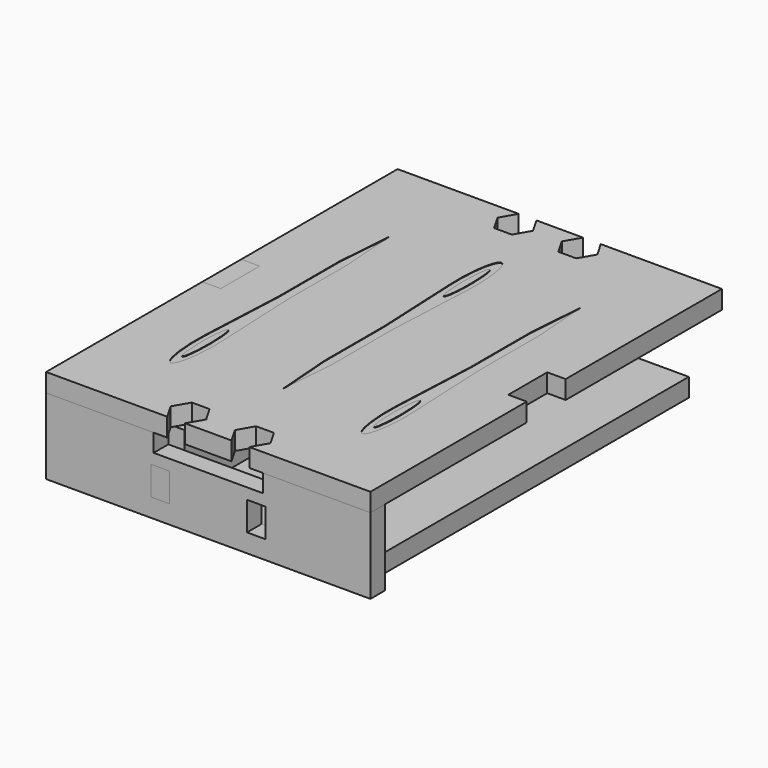
from build123d import *

# Parameters (mm, degrees)
F1_W      = 50
F1_H      = 70
F1_W_2    = 3.2
F1_H_2    = 23.3333333333
F2_DEPTH  = 3.2
F4_DEPTH  = 3.2
F6_DEPTH  = 3.2
F8_DEPTH  = 3.2
F10_DEPTH = 3.2
F11_W     = 18.7
F11_H     = 3.2
F12_DEPTH = 3.2
F14_DEPTH = 0.1
F16_DEPTH = 3.2


# Not quite as in the source:
# - a feature names something its author has since deleted; it is built from what else it names


with BuildPart() as f2:
    # F1 (on Top) → F2 (new body)
    with BuildSketch(Plane.XY):
        Rectangle(F1_W, F1_H)
        with Locations((-8.3333333333, 0)):
            Rectangle(F1_W_2, F1_H_2, mode=Mode.SUBTRACT)
        with Locations((8.3333333333, 0)):
            Rectangle(F1_W_2, F1_H_2, mode=Mode.SUBTRACT)
    extrude(amount=F2_DEPTH)


with BuildPart() as f4:
    # F3 (on face) → F4 (new body)
    with BuildSketch(Plane(origin=(-25, 0, 0), x_dir=(0, -1, 0), z_dir=(-1, 0, 0))):
        Polygon((-35, 13.2), (-35, 0), (35, 0), (35, 13.2), (14.2401693586, 13.2), (8.4666666667, 3.2), (-8.4666666667, 3.2), (-14.2401693586, 13.2), align=None)
    extrude(amount=F4_DEPTH)


with BuildPart() as f6:
    # F5 (on face) → F6 (new body)
    with BuildSketch(Plane(origin=(-6.7333333333, 0, 0), x_dir=(0, -1, 0), z_dir=(-1, 0, 0))):
        Polygon((38.2, 3.2), (38.2, 8.2), (35, 8.2), (35, 13.2), (14.2401693586, 13.2), (8.4666666667, 3.2), (11.6666666667, 3.2), (35, 3.2), align=None)
        Polygon((-8.4666666667, 3.2), (-14.2401693586, 13.2), (-35, 13.2), (-35, 8.2), (-38.2, 8.2), (-38.2, 3.2), (-35, 3.2), (-11.6666666667, 3.2), align=None)
        Polygon((11.6666666667, 0), (11.6666666667, 3.2), (8.4666666667, 3.2), (-8.4666666667, 3.2), (-11.6666666667, 3.2), (-11.6666666667, 0), align=None)
    extrude(amount=F6_DEPTH)


with BuildPart() as f8:
    # F7 (on face) → F8 (new body)
    with BuildSketch(Plane.XZ.offset(35)):
        Polygon((25, 3.2), (25, 0), (28.2, 0), (28.2, 13.2), (25, 13.2), align=None)
        Polygon((-25, 3.2), (-25, 0), (25, 0), (25, 3.2), (9.9333333333, 3.2), (6.7333333333, 3.2), (-6.7333333333, 3.2), (-9.9333333333, 3.2), align=None)
        Polygon((-28.2, 13.2), (-28.2, 0), (-25, 0), (-25, 3.2), (-9.9333333333, 3.2), (-9.9333333333, 8.2), (-6.7333333333, 8.2), (-6.7333333333, 3.2), (6.7333333333, 3.2), (6.7333333333, 8.2), (9.9333333333, 8.2), (9.9333333333, 3.2), (25, 3.2), (25, 13.2), (9.5, 13.2), (9.5, 10.1), (-9.5, 10.1), (-9.5, 13.2), align=None)
    extrude(amount=F8_DEPTH)


with BuildPart() as f10:
    # F9 (on face) → F10 (new body)
    with BuildSketch(Plane(origin=(-28.2, 0, 0), x_dir=(0, -1, 0), z_dir=(-1, 0, 0))):
        Polygon((-14.2401693586, 13.2), (-8.4666666667, 3.2), (8.4666666667, 3.2), (14.2401693586, 13.2), (4.2333333333, 13.2), (4.2333333333, 16.4), (-4.2333333333, 16.4), (-4.2333333333, 13.2), align=None)
    extrude(amount=-F10_DEPTH)


with BuildPart() as f12:
    # F11 (on face) → F12 (new body)
    with BuildSketch(Plane.XY.offset(13.2)):
        Polygon((-28.2, 38.2), (-28.2, 4.2333333333), (-25, 4.2333333333), (-25, -4.2333333333), (-28.2, -4.2333333333), (-28.2, -35), (-9.5, -35), (-9.5, -38.2), (-7.1332359102, -38.2), (-8.6776478803, -35.525), (-7.1332359102, -32.85), (-4.0444119701, -32.85), (-2.5, -35.525), (-4.0444119701, -38.2), (4.0444119701, -38.2), (2.5, -35.525), (4.0444119701, -32.85), (7.1332359102, -32.85), (8.6776478803, -35.525), (7.1332359102, -38.2), (9.5, -38.2), (9.5, -35), (28.2, -35), (28.2, -4.2333333333), (25, -4.2333333333), (25, 4.2333333333), (28.2, 4.2333333333), (28.2, 38.2), (7.1332359102, 38.2), (8.6776478803, 35.525), (7.1332359102, 32.85), (4.0444119701, 32.85), (2.5, 35.525), (4.0444119701, 38.2), (-4.0444119701, 38.2), (-2.5, 35.525), (-4.0444119701, 32.85), (-7.1332359102, 32.85), (-8.6776478803, 35.525), (-7.1332359102, 38.2), align=None)
        with Locations((-18.85, -36.6)):
            Rectangle(F11_W, F11_H)
        with Locations((18.85, -36.6)):
            Rectangle(F11_W, F11_H)
    extrude(amount=F12_DEPTH)

    # F13 (on face) → F14 (cut)
    with BuildSketch(Plane.XY.offset(16.4)):
        with BuildLine():
            add(Edge.make_bspline(
                [(-18.1277491736, -16.3026645297), (-18.5551299314, -25.5), (-16.6666666667, -25.5)],
                knots=[4.4840998278, 4.4840998278, 4.4840998278, 6.2831853072, 6.2831853072, 6.2831853072], degree=2, weights=[1, 0.6219680876, 1]))
            add(Edge.make_bspline(
                [(-16.6666666667, -25.5), (-14.7782034019, -25.5), (-15.2055841597, -16.3026645297)],
                knots=[0, 0, 0, 1.7990854794, 1.7990854794, 1.7990854794], degree=2, weights=[1, 0.6219680876, 1]))
            add(Edge.make_bspline(
                [(-15.2055841597, -16.3026645297), (-15.4752217273, -10.5), (-16.6666666667, -10.5), (-17.8581116061, -10.5), (-18.1277491736, -16.3026645297)],
                knots=[1.7990854794, 1.7990854794, 1.7990854794, 3.1415926536, 3.1415926536, 4.4840998278, 4.4840998278, 4.4840998278], degree=2, weights=[1, 0.7830425902, 1, 0.7830425902, 1]))
        make_face()
        with BuildLine():
            add(Edge.make_bspline(
                [(-16.6666666667, -23), (-15.6274361821, -23), (-16.1470514244, -15.5), (-16.6666666667, -8), (-17.1862819089, -15.5), (-17.7058971512, -23), (-16.6666666667, -23)],
                knots=[0, 0, 0, 2.0943951024, 2.0943951024, 4.1887902048, 4.1887902048, 6.2831853072, 6.2831853072, 6.2831853072], degree=2, weights=[1, 0.5, 1, 0.5, 1, 0.5, 1]))
        make_face(mode=Mode.SUBTRACT)
        with BuildLine():
            add(Edge.make_bspline(
                [(-15.2055841597, -16.3026645297), (-15.4752217273, -10.5), (-16.6666666667, -10.5), (-17.8581116061, -10.5), (-18.1277491736, -16.3026645297)],
                knots=[1.7990854794, 1.7990854794, 1.7990854794, 3.1415926536, 3.1415926536, 4.4840998278, 4.4840998278, 4.4840998278], degree=2, weights=[1, 0.7830425902, 1, 0.7830425902, 1]))
            Line((-15.2055841597, -16.3026645297), (-15.9166666667, -1))
            Line((-15.9166666667, -1), (-15.9166666667, 12.0281646624))
            Line((-15.9166666667, 12.0281646624), (-16.6666666667, 22))
            Line((-16.6666666667, 22), (-17.4166666667, 12.0281646624))
            Line((-17.4166666667, 12.0281646624), (-17.4166666667, -1))
            Line((-17.4166666667, -1), (-18.1277491736, -16.3026645297))
        make_face()
        with BuildLine():
            Line((-1.4610825069, 16.3026645297), (-0.75, 1))
            Line((-0.75, 1), (-0.75, -12.0281646624))
            Line((-0.75, -12.0281646624), (0, -22))
            Line((0, -22), (0.75, -12.0281646624))
            Line((0.75, -12.0281646624), (0.75, 1))
            Line((0.75, 1), (1.4610825069, 16.3026645297))
            add(Edge.make_bspline(
                [(-1.4610825069, 16.3026645297), (-1.1914449394, 10.5), (0, 10.5), (1.1914449394, 10.5), (1.4610825069, 16.3026645297)],
                knots=[1.7990854794, 1.7990854794, 1.7990854794, 3.1415926536, 3.1415926536, 4.4840998278, 4.4840998278, 4.4840998278], degree=2, weights=[1, 0.7830425902, 1, 0.7830425902, 1]))
        make_face()
        with BuildLine():
            add(Edge.make_bspline(
                [(0, 25.5), (-1.8884632647, 25.5), (-1.4610825069, 16.3026645297)],
                knots=[0, 0, 0, 1.7990854794, 1.7990854794, 1.7990854794], degree=2, weights=[1, 0.6219680876, 1]))
            add(Edge.make_bspline(
                [(-1.4610825069, 16.3026645297), (-1.1914449394, 10.5), (0, 10.5), (1.1914449394, 10.5), (1.4610825069, 16.3026645297)],
                knots=[1.7990854794, 1.7990854794, 1.7990854794, 3.1415926536, 3.1415926536, 4.4840998278, 4.4840998278, 4.4840998278], degree=2, weights=[1, 0.7830425902, 1, 0.7830425902, 1]))
            add(Edge.make_bspline(
                [(1.4610825069, 16.3026645297), (1.8884632647, 25.5), (0, 25.5)],
                knots=[4.4840998278, 4.4840998278, 4.4840998278, 6.2831853072, 6.2831853072, 6.2831853072], degree=2, weights=[1, 0.6219680876, 1]))
        make_face()
        with BuildLine():
            add(Edge.make_bspline(
                [(0, 23), (-1.0392304845, 23), (-0.5196152423, 15.5), (0, 8), (0.5196152423, 15.5), (1.0392304845, 23), (0, 23)],
                knots=[0, 0, 0, 2.0943951024, 2.0943951024, 4.1887902048, 4.1887902048, 6.2831853072, 6.2831853072, 6.2831853072], degree=2, weights=[1, 0.5, 1, 0.5, 1, 0.5, 1]))
        make_face(mode=Mode.SUBTRACT)
        with BuildLine():
            Line((18.1277491736, -16.3026645297), (17.4166666667, -1))
            Line((17.4166666667, -1), (17.4166666667, 12.0281646624))
            Line((17.4166666667, 12.0281646624), (16.6666666667, 22))
            Line((16.6666666667, 22), (15.9166666667, 12.0281646624))
            Line((15.9166666667, 12.0281646624), (15.9166666667, -1))
            Line((15.9166666667, -1), (15.2055841597, -16.3026645297))
            add(Edge.make_bspline(
                [(18.1277491736, -16.3026645297), (17.8581116061, -10.5), (16.6666666667, -10.5), (15.4752217273, -10.5), (15.2055841597, -16.3026645297)],
                knots=[1.7990854794, 1.7990854794, 1.7990854794, 3.1415926536, 3.1415926536, 4.4840998278, 4.4840998278, 4.4840998278], degree=2, weights=[1, 0.7830425902, 1, 0.7830425902, 1]))
        make_face()
        with BuildLine():
            add(Edge.make_bspline(
                [(16.6666666667, -25.5), (18.5551299314, -25.5), (18.1277491736, -16.3026645297)],
                knots=[0, 0, 0, 1.7990854794, 1.7990854794, 1.7990854794], degree=2, weights=[1, 0.6219680876, 1]))
            add(Edge.make_bspline(
                [(18.1277491736, -16.3026645297), (17.8581116061, -10.5), (16.6666666667, -10.5), (15.4752217273, -10.5), (15.2055841597, -16.3026645297)],
                knots=[1.7990854794, 1.7990854794, 1.7990854794, 3.1415926536, 3.1415926536, 4.4840998278, 4.4840998278, 4.4840998278], degree=2, weights=[1, 0.7830425902, 1, 0.7830425902, 1]))
            add(Edge.make_bspline(
                [(15.2055841597, -16.3026645297), (14.7782034019, -25.5), (16.6666666667, -25.5)],
                knots=[4.4840998278, 4.4840998278, 4.4840998278, 6.2831853072, 6.2831853072, 6.2831853072], degree=2, weights=[1, 0.6219680876, 1]))
        make_face()
        with BuildLine():
            add(Edge.make_bspline(
                [(16.6666666667, -23), (17.7058971512, -23), (17.1862819089, -15.5), (16.6666666667, -8), (16.1470514244, -15.5), (15.6274361821, -23), (16.6666666667, -23)],
                knots=[0, 0, 0, 2.0943951024, 2.0943951024, 4.1887902048, 4.1887902048, 6.2831853072, 6.2831853072, 6.2831853072], degree=2, weights=[1, 0.5, 1, 0.5, 1, 0.5, 1]))
        make_face(mode=Mode.SUBTRACT)
    extrude(amount=-F14_DEPTH, mode=Mode.SUBTRACT)


with BuildPart() as f16:
    # F15 (on face) → F16 (new body)
    with BuildSketch(Plane.XY.offset(13.2)):
        Polygon((-22.5, 16.75), (-24.5, 16.75), (-24.5, 8.75), (-25, 8.75), (-25, -8.75), (-24.5, -8.75), (-24.5, -16.75), (-22.5, -16.75), align=None)
    extrude(amount=-F16_DEPTH)


solid = Compound([f2.part, f4.part, f6.part, f8.part, f10.part, f12.part, f16.part])
